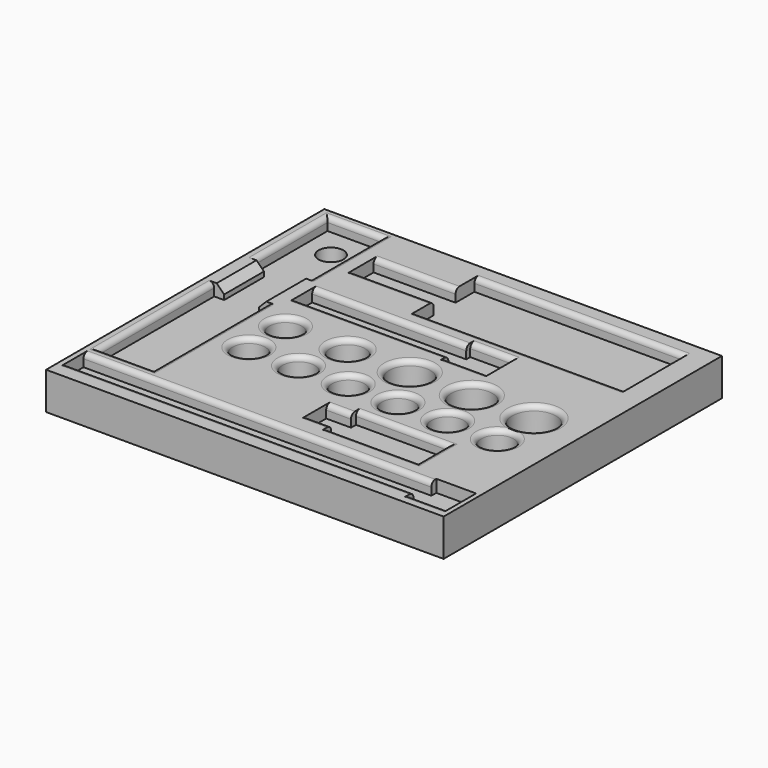
from build123d import *

# Parameters (mm, degrees)
F0_W          = 160
F0_H          = 140
F0_R          = 6.5
F0_R_2        = 7
F0_R_3        = 8.25
F0_R_4        = 8.75
F0_R_5        = 5
F1_DEPTH      = 1
F2_DEPTH      = 10
F3_DEPTH      = 15
F4_SIZE       = 3
F5_T1_DEPTH   = 37
F5_T3_DEPTH   = 58
F5_T5_DEPTH   = 22
F5_T7_DEPTH   = 145
F5_T9_DEPTH   = 16
F5_T11_DEPTH  = 85
F5_T13_DEPTH  = 38
F5_T15_DEPTH  = 18
F5_T17_DEPTH  = 67
F5_T19_DEPTH  = 37
F5_T21_DEPTH  = 15
F5_T23_DEPTH  = 15
F5_T51_DEPTH  = 27
F5_T56_DEPTH  = 42
F5_T64_DEPTH  = 42
F5_T69_DEPTH  = 27
F5_T76_DEPTH  = 63
F5_T80_DEPTH  = 27
F5_T87_DEPTH  = 27
F5_T92_DEPTH  = 63
F5_T99_DEPTH  = 42
F5_T103_DEPTH = 20
F5_T110_DEPTH = 20
F5_T114_DEPTH = 42


# Not quite as in the source:
# - a fillet or chamfer that OpenCascade refuses, or shapes differently, is made with other operations: its cross-section is extruded or revolved along the edge and cut away or added
# - a feature names something its author has since deleted; it is built from what else it names


with BuildPart() as f1:
    # F0 (on Top) → F1 (new body)
    with BuildSketch(Plane.XY):
        Rectangle(F0_W, F0_H)
        with Locations((-39.7392310202, -18.3150917292)):
            Circle(F0_R, mode=Mode.SUBTRACT)
        with Locations((-19.7392310202, -18.3150917292)):
            Circle(F0_R, mode=Mode.SUBTRACT)
        Polygon((78.1284613013, -51.3328099847), (78.1284613013, -65.3328099847), (62.1284613013, -65.3328099847), (62.1284613013, -62.8328099847), (-77.8715386987, -62.8328099847), (-77.8715386987, -53.8328099847), (62.1284613013, -53.8328099847), (62.1284613013, -51.3328099847), align=None, mode=Mode.SUBTRACT)
        Polygon((3.4841548279, -43.4470043983), (3.4841548279, -33.4470043983), (13.4841548279, -33.4470043983), (13.4841548279, -30.9470043983), (50.4841548279, -30.9470043983), (50.4841548279, -45.9470043983), (13.4841548279, -45.9470043983), (13.4841548279, -43.4470043983), align=None, mode=Mode.SUBTRACT)
        with Locations((0.2607689798, -18.3150917292)):
            Circle(F0_R, mode=Mode.SUBTRACT)
        with Locations((20.2607689798, -18.3150917292)):
            Circle(F0_R, mode=Mode.SUBTRACT)
        with Locations((40.2607689798, -18.3150917292)):
            Circle(F0_R, mode=Mode.SUBTRACT)
        with Locations((60.2607689798, -18.3150917292)):
            Circle(F0_R, mode=Mode.SUBTRACT)
        Polygon((-75.9079491794, 29.4701200724), (-75.9079491794, 66.4701200724), (-53.9079491794, 66.4701200724), (-53.9079491794, 29.4701200724), (-57.9079491794, 29.4701200724), (-57.9079491794, 9.4701200724), (-53.9079491794, 9.4701200724), (-53.9079491794, -48.5298799276), (-75.9079491794, -48.5298799276), (-75.9079491794, 9.4701200724), (-71.9079491794, 9.4701200724), (-71.9079491794, 29.4701200724), align=None, mode=Mode.SUBTRACT)
        with Locations((-39.6466106176, 0)):
            Circle(F0_R, mode=Mode.SUBTRACT)
        with Locations((-14.6466106176, 0)):
            Circle(F0_R_2, mode=Mode.SUBTRACT)
        Polygon((30.7263465822, 27.4683196438), (30.7263465822, 14.4683196438), (12.7263465822, 14.4683196438), (12.7263465822, 16.4683196438), (-49.2736534178, 16.4683196438), (-49.2736534178, 25.4683196438), (12.7263465822, 25.4683196438), (12.7263465822, 27.4683196438), align=None, mode=Mode.SUBTRACT)
        with Locations((10.3533893824, 0)):
            Circle(F0_R_3, mode=Mode.SUBTRACT)
        with Locations((35.3533893824, 0)):
            Circle(F0_R_3, mode=Mode.SUBTRACT)
        with Locations((60.3533893824, 0)):
            Circle(F0_R_4, mode=Mode.SUBTRACT)
        Polygon((71.00115427, 62.9950422049), (71.00115427, 32.9950422049), (-13.99884573, 32.9950422049), (-13.99884573, 42.4950422049), (-46.99884573, 42.4950422049), (-46.99884573, 53.4950422049), (-13.99884573, 53.4950422049), (-13.99884573, 62.9950422049), align=None, mode=Mode.SUBTRACT)
        Polygon((-13.99884573, 32.9950422049), (71.00115427, 32.9950422049), (71.00115427, 62.9950422049), (-13.99884573, 62.9950422049), (-13.99884573, 53.4950422049), (-46.99884573, 53.4950422049), (-46.99884573, 42.4950422049), (-13.99884573, 42.4950422049), align=None)
        Polygon((-53.9079491794, 66.4701200724), (-75.9079491794, 66.4701200724), (-75.9079491794, 29.4701200724), (-71.9079491794, 29.4701200724), (-71.9079491794, 9.4701200724), (-75.9079491794, 9.4701200724), (-75.9079491794, -48.5298799276), (-53.9079491794, -48.5298799276), (-53.9079491794, 9.4701200724), (-57.9079491794, 9.4701200724), (-57.9079491794, 29.4701200724), (-53.9079491794, 29.4701200724), align=None)
        with Locations((-64.9079491794, 54.4701200724)):
            Circle(F0_R_5, mode=Mode.SUBTRACT)
        Polygon((62.1284613013, -65.3328099847), (78.1284613013, -65.3328099847), (78.1284613013, -51.3328099847), (62.1284613013, -51.3328099847), (62.1284613013, -53.8328099847), (-77.8715386987, -53.8328099847), (-77.8715386987, -62.8328099847), (62.1284613013, -62.8328099847), align=None)
        Polygon((12.7263465822, 14.4683196438), (30.7263465822, 14.4683196438), (30.7263465822, 27.4683196438), (12.7263465822, 27.4683196438), (12.7263465822, 25.4683196438), (-49.2736534178, 25.4683196438), (-49.2736534178, 16.4683196438), (12.7263465822, 16.4683196438), align=None)
        Polygon((13.4841548279, -33.4470043983), (3.4841548279, -33.4470043983), (3.4841548279, -43.4470043983), (13.4841548279, -43.4470043983), (13.4841548279, -45.9470043983), (50.4841548279, -45.9470043983), (50.4841548279, -30.9470043983), (13.4841548279, -30.9470043983), align=None)
        with Locations((60.3533893824, 0)):
            Circle(F0_R_4)
        with Locations((10.3533893824, 0)):
            Circle(F0_R_3)
        with Locations((35.3533893824, 0)):
            Circle(F0_R_3)
        with Locations((-14.6466106176, 0)):
            Circle(F0_R_2)
        with Locations((-39.6466106176, 0)):
            Circle(F0_R)
        with Locations((-39.7392310202, -18.3150917292)):
            Circle(F0_R)
        with Locations((-19.7392310202, -18.3150917292)):
            Circle(F0_R)
        with Locations((0.2607689798, -18.3150917292)):
            Circle(F0_R)
        with Locations((20.2607689798, -18.3150917292)):
            Circle(F0_R)
        with Locations((40.2607689798, -18.3150917292)):
            Circle(F0_R)
        with Locations((60.2607689798, -18.3150917292)):
            Circle(F0_R)
        with Locations((-64.9079491794, 54.4701200724)):
            Circle(F0_R_5)
    extrude(amount=F1_DEPTH)

    # F0 (on Top) → F2 (join)
    with BuildSketch(Plane.XY):
        Rectangle(F0_W, F0_H)
        with Locations((-39.7392310202, -18.3150917292)):
            Circle(F0_R, mode=Mode.SUBTRACT)
        with Locations((-19.7392310202, -18.3150917292)):
            Circle(F0_R, mode=Mode.SUBTRACT)
        Polygon((78.1284613013, -51.3328099847), (78.1284613013, -65.3328099847), (62.1284613013, -65.3328099847), (62.1284613013, -62.8328099847), (-77.8715386987, -62.8328099847), (-77.8715386987, -53.8328099847), (62.1284613013, -53.8328099847), (62.1284613013, -51.3328099847), align=None, mode=Mode.SUBTRACT)
        Polygon((3.4841548279, -43.4470043983), (3.4841548279, -33.4470043983), (13.4841548279, -33.4470043983), (13.4841548279, -30.9470043983), (50.4841548279, -30.9470043983), (50.4841548279, -45.9470043983), (13.4841548279, -45.9470043983), (13.4841548279, -43.4470043983), align=None, mode=Mode.SUBTRACT)
        with Locations((0.2607689798, -18.3150917292)):
            Circle(F0_R, mode=Mode.SUBTRACT)
        with Locations((20.2607689798, -18.3150917292)):
            Circle(F0_R, mode=Mode.SUBTRACT)
        with Locations((40.2607689798, -18.3150917292)):
            Circle(F0_R, mode=Mode.SUBTRACT)
        with Locations((60.2607689798, -18.3150917292)):
            Circle(F0_R, mode=Mode.SUBTRACT)
        Polygon((-75.9079491794, 29.4701200724), (-75.9079491794, 66.4701200724), (-53.9079491794, 66.4701200724), (-53.9079491794, 29.4701200724), (-57.9079491794, 29.4701200724), (-57.9079491794, 9.4701200724), (-53.9079491794, 9.4701200724), (-53.9079491794, -48.5298799276), (-75.9079491794, -48.5298799276), (-75.9079491794, 9.4701200724), (-71.9079491794, 9.4701200724), (-71.9079491794, 29.4701200724), align=None, mode=Mode.SUBTRACT)
        with Locations((-39.6466106176, 0)):
            Circle(F0_R, mode=Mode.SUBTRACT)
        with Locations((-14.6466106176, 0)):
            Circle(F0_R_2, mode=Mode.SUBTRACT)
        Polygon((30.7263465822, 27.4683196438), (30.7263465822, 14.4683196438), (12.7263465822, 14.4683196438), (12.7263465822, 16.4683196438), (-49.2736534178, 16.4683196438), (-49.2736534178, 25.4683196438), (12.7263465822, 25.4683196438), (12.7263465822, 27.4683196438), align=None, mode=Mode.SUBTRACT)
        with Locations((10.3533893824, 0)):
            Circle(F0_R_3, mode=Mode.SUBTRACT)
        with Locations((35.3533893824, 0)):
            Circle(F0_R_3, mode=Mode.SUBTRACT)
        with Locations((60.3533893824, 0)):
            Circle(F0_R_4, mode=Mode.SUBTRACT)
        Polygon((71.00115427, 62.9950422049), (71.00115427, 32.9950422049), (-13.99884573, 32.9950422049), (-13.99884573, 42.4950422049), (-46.99884573, 42.4950422049), (-46.99884573, 53.4950422049), (-13.99884573, 53.4950422049), (-13.99884573, 62.9950422049), align=None, mode=Mode.SUBTRACT)
        Polygon((62.1284613013, -65.3328099847), (78.1284613013, -65.3328099847), (78.1284613013, -51.3328099847), (62.1284613013, -51.3328099847), (62.1284613013, -53.8328099847), (-77.8715386987, -53.8328099847), (-77.8715386987, -62.8328099847), (62.1284613013, -62.8328099847), align=None)
        Polygon((-53.9079491794, 66.4701200724), (-75.9079491794, 66.4701200724), (-75.9079491794, 29.4701200724), (-71.9079491794, 29.4701200724), (-71.9079491794, 9.4701200724), (-75.9079491794, 9.4701200724), (-75.9079491794, -48.5298799276), (-53.9079491794, -48.5298799276), (-53.9079491794, 9.4701200724), (-57.9079491794, 9.4701200724), (-57.9079491794, 29.4701200724), (-53.9079491794, 29.4701200724), align=None)
        with Locations((-64.9079491794, 54.4701200724)):
            Circle(F0_R_5, mode=Mode.SUBTRACT)
        Polygon((12.7263465822, 14.4683196438), (30.7263465822, 14.4683196438), (30.7263465822, 27.4683196438), (12.7263465822, 27.4683196438), (12.7263465822, 25.4683196438), (-49.2736534178, 25.4683196438), (-49.2736534178, 16.4683196438), (12.7263465822, 16.4683196438), align=None)
        Polygon((13.4841548279, -33.4470043983), (3.4841548279, -33.4470043983), (3.4841548279, -43.4470043983), (13.4841548279, -43.4470043983), (13.4841548279, -45.9470043983), (50.4841548279, -45.9470043983), (50.4841548279, -30.9470043983), (13.4841548279, -30.9470043983), align=None)
        Polygon((-13.99884573, 32.9950422049), (71.00115427, 32.9950422049), (71.00115427, 62.9950422049), (-13.99884573, 62.9950422049), (-13.99884573, 53.4950422049), (-46.99884573, 53.4950422049), (-46.99884573, 42.4950422049), (-13.99884573, 42.4950422049), align=None)
    extrude(amount=F2_DEPTH)

    # F0 (on Top) → F3 (join)
    with BuildSketch(Plane.XY):
        Rectangle(F0_W, F0_H)
        with Locations((-39.7392310202, -18.3150917292)):
            Circle(F0_R, mode=Mode.SUBTRACT)
        with Locations((-19.7392310202, -18.3150917292)):
            Circle(F0_R, mode=Mode.SUBTRACT)
        Polygon((78.1284613013, -51.3328099847), (78.1284613013, -65.3328099847), (62.1284613013, -65.3328099847), (62.1284613013, -62.8328099847), (-77.8715386987, -62.8328099847), (-77.8715386987, -53.8328099847), (62.1284613013, -53.8328099847), (62.1284613013, -51.3328099847), align=None, mode=Mode.SUBTRACT)
        Polygon((3.4841548279, -43.4470043983), (3.4841548279, -33.4470043983), (13.4841548279, -33.4470043983), (13.4841548279, -30.9470043983), (50.4841548279, -30.9470043983), (50.4841548279, -45.9470043983), (13.4841548279, -45.9470043983), (13.4841548279, -43.4470043983), align=None, mode=Mode.SUBTRACT)
        with Locations((0.2607689798, -18.3150917292)):
            Circle(F0_R, mode=Mode.SUBTRACT)
        with Locations((20.2607689798, -18.3150917292)):
            Circle(F0_R, mode=Mode.SUBTRACT)
        with Locations((40.2607689798, -18.3150917292)):
            Circle(F0_R, mode=Mode.SUBTRACT)
        with Locations((60.2607689798, -18.3150917292)):
            Circle(F0_R, mode=Mode.SUBTRACT)
        Polygon((-75.9079491794, 29.4701200724), (-75.9079491794, 66.4701200724), (-53.9079491794, 66.4701200724), (-53.9079491794, 29.4701200724), (-57.9079491794, 29.4701200724), (-57.9079491794, 9.4701200724), (-53.9079491794, 9.4701200724), (-53.9079491794, -48.5298799276), (-75.9079491794, -48.5298799276), (-75.9079491794, 9.4701200724), (-71.9079491794, 9.4701200724), (-71.9079491794, 29.4701200724), align=None, mode=Mode.SUBTRACT)
        with Locations((-39.6466106176, 0)):
            Circle(F0_R, mode=Mode.SUBTRACT)
        with Locations((-14.6466106176, 0)):
            Circle(F0_R_2, mode=Mode.SUBTRACT)
        Polygon((30.7263465822, 27.4683196438), (30.7263465822, 14.4683196438), (12.7263465822, 14.4683196438), (12.7263465822, 16.4683196438), (-49.2736534178, 16.4683196438), (-49.2736534178, 25.4683196438), (12.7263465822, 25.4683196438), (12.7263465822, 27.4683196438), align=None, mode=Mode.SUBTRACT)
        with Locations((10.3533893824, 0)):
            Circle(F0_R_3, mode=Mode.SUBTRACT)
        with Locations((35.3533893824, 0)):
            Circle(F0_R_3, mode=Mode.SUBTRACT)
        with Locations((60.3533893824, 0)):
            Circle(F0_R_4, mode=Mode.SUBTRACT)
        Polygon((71.00115427, 62.9950422049), (71.00115427, 32.9950422049), (-13.99884573, 32.9950422049), (-13.99884573, 42.4950422049), (-46.99884573, 42.4950422049), (-46.99884573, 53.4950422049), (-13.99884573, 53.4950422049), (-13.99884573, 62.9950422049), align=None, mode=Mode.SUBTRACT)
    extrude(amount=F3_DEPTH)

    # F4
    f4_edges = [f1.edges().sort_by_distance(p)[0] for p in [
        (-57.907949, 19.47012, 15),
        (-71.907949, 19.47012, 15),
    ]]
    chamfer(f4_edges, length=F4_SIZE)

    # F5: fillet of radius 2 on 33 edges, made by hand

    # F5_s2 → F5_t1 (cut)
    with BuildSketch(Plane.XZ.offset(-66.4701200724)):
        with BuildLine():
            ThreePointArc((-77.9079491794, 15), (-76.493735617, 14.4142135624), (-75.9079491794, 13))
            Line((-75.9079491794, 13), (-75.9079491794, 15))
            Line((-75.9079491794, 15), (-77.9079491794, 15))
        make_face()
        with BuildLine():
            ThreePointArc((-51.9079491794, 15), (-53.3221627418, 14.4142135624), (-53.9079491794, 13))
            Line((-53.9079491794, 13), (-53.9079491794, 15))
            Line((-53.9079491794, 15), (-51.9079491794, 15))
        make_face()
    extrude(amount=F5_T1_DEPTH, mode=Mode.SUBTRACT)

    # F5_s4 → F5_t3 (cut)
    with BuildSketch(Plane.XZ.offset(-9.4701200724)):
        with BuildLine():
            ThreePointArc((-51.9079491794, 15), (-53.3221627418, 14.4142135624), (-53.9079491794, 13))
            Line((-53.9079491794, 13), (-53.9079491794, 15))
            Line((-53.9079491794, 15), (-51.9079491794, 15))
        make_face()
        with BuildLine():
            ThreePointArc((-77.9079491794, 15), (-76.493735617, 14.4142135624), (-75.9079491794, 13))
            Line((-75.9079491794, 13), (-75.9079491794, 15))
            Line((-75.9079491794, 15), (-77.9079491794, 15))
        make_face()
    extrude(amount=F5_T3_DEPTH, mode=Mode.SUBTRACT)

    # F5_s6 → F5_t5 (cut)
    with BuildSketch(Plane.YZ.offset(-75.9079491794)):
        with BuildLine():
            ThreePointArc((-50.5298799276, 15), (-49.1156663653, 14.4142135624), (-48.5298799276, 13))
            Line((-48.5298799276, 13), (-48.5298799276, 15))
            Line((-48.5298799276, 15), (-50.5298799276, 15))
        make_face()
        with BuildLine():
            ThreePointArc((68.4701200724, 15), (67.05590651, 14.4142135624), (66.4701200724, 13))
            Line((66.4701200724, 13), (66.4701200724, 15))
            Line((66.4701200724, 15), (68.4701200724, 15))
        make_face()
    extrude(amount=F5_T5_DEPTH, mode=Mode.SUBTRACT)

    # F5_s8 → F5_t7 (cut)
    with BuildSketch(Plane.YZ.offset(-77.8715386987)):
        with BuildLine():
            ThreePointArc((-64.8328099847, 15), (-63.4185964223, 14.4142135624), (-62.8328099847, 13))
            Line((-62.8328099847, 13), (-62.8328099847, 15))
            Line((-62.8328099847, 15), (-64.8328099847, 15))
        make_face()
        with BuildLine():
            ThreePointArc((-51.8328099847, 15), (-53.2470235471, 14.4142135624), (-53.8328099847, 13))
            Line((-53.8328099847, 13), (-53.8328099847, 15))
            Line((-53.8328099847, 15), (-51.8328099847, 15))
        make_face()
    extrude(amount=F5_T7_DEPTH, mode=Mode.SUBTRACT)

    # F5_s10 → F5_t9 (cut)
    with BuildSketch(Plane.YZ.offset(62.1284613013)):
        with BuildLine():
            ThreePointArc((-67.3328099847, 15), (-65.9185964223, 14.4142135624), (-65.3328099847, 13))
            Line((-65.3328099847, 13), (-65.3328099847, 15))
            Line((-65.3328099847, 15), (-67.3328099847, 15))
        make_face()
    extrude(amount=F5_T9_DEPTH, mode=Mode.SUBTRACT)

    # F5_s12 → F5_t11 (cut)
    with BuildSketch(Plane.YZ.offset(-13.99884573)):
        with BuildLine():
            ThreePointArc((64.9950422049, 15), (63.5808286425, 14.4142135624), (62.9950422049, 13))
            Line((62.9950422049, 13), (62.9950422049, 15))
            Line((62.9950422049, 15), (64.9950422049, 15))
        make_face()
        with BuildLine():
            ThreePointArc((30.9950422049, 15), (32.4092557672, 14.4142135624), (32.9950422049, 13))
            Line((32.9950422049, 13), (32.9950422049, 15))
            Line((32.9950422049, 15), (30.9950422049, 15))
        make_face()
    extrude(amount=F5_T11_DEPTH, mode=Mode.SUBTRACT)

    # F5_s14 → F5_t13 (cut)
    with BuildSketch(Plane.YZ.offset(-46.99884573)):
        with BuildLine():
            ThreePointArc((40.4950422049, 15), (41.9092557672, 14.4142135624), (42.4950422049, 13))
            Line((42.4950422049, 13), (42.4950422049, 15))
            Line((42.4950422049, 15), (40.4950422049, 15))
        make_face()
        with BuildLine():
            ThreePointArc((55.4950422049, 15), (54.0808286425, 14.4142135624), (53.4950422049, 13))
            Line((53.4950422049, 13), (53.4950422049, 15))
            Line((53.4950422049, 15), (55.4950422049, 15))
        make_face()
    extrude(amount=F5_T13_DEPTH, mode=Mode.SUBTRACT)

    # F5_s16 → F5_t15 (cut)
    with BuildSketch(Plane.YZ.offset(12.7263465822)):
        with BuildLine():
            ThreePointArc((29.4683196438, 15), (28.0541060814, 14.4142135624), (27.4683196438, 13))
            Line((27.4683196438, 13), (27.4683196438, 15))
            Line((27.4683196438, 15), (29.4683196438, 15))
        make_face()
        with BuildLine():
            ThreePointArc((12.4683196438, 15), (13.8825332061, 14.4142135624), (14.4683196438, 13))
            Line((14.4683196438, 13), (14.4683196438, 15))
            Line((14.4683196438, 15), (12.4683196438, 15))
        make_face()
    extrude(amount=F5_T15_DEPTH, mode=Mode.SUBTRACT)

    # F5_s18 → F5_t17 (cut)
    with BuildSketch(Plane.YZ.offset(-49.2736534178)):
        with BuildLine():
            ThreePointArc((14.4683196438, 15), (15.8825332061, 14.4142135624), (16.4683196438, 13))
            Line((16.4683196438, 13), (16.4683196438, 15))
            Line((16.4683196438, 15), (14.4683196438, 15))
        make_face()
        with BuildLine():
            ThreePointArc((27.4683196438, 15), (26.0541060814, 14.4142135624), (25.4683196438, 13))
            Line((25.4683196438, 13), (25.4683196438, 15))
            Line((25.4683196438, 15), (27.4683196438, 15))
        make_face()
    extrude(amount=F5_T17_DEPTH, mode=Mode.SUBTRACT)

    # F5_s20 → F5_t19 (cut)
    with BuildSketch(Plane.YZ.offset(13.4841548279)):
        with BuildLine():
            ThreePointArc((-28.9470043983, 15), (-30.3612179607, 14.4142135624), (-30.9470043983, 13))
            Line((-30.9470043983, 13), (-30.9470043983, 15))
            Line((-30.9470043983, 15), (-28.9470043983, 15))
        make_face()
        with BuildLine():
            ThreePointArc((-47.9470043983, 15), (-46.532790836, 14.4142135624), (-45.9470043983, 13))
            Line((-45.9470043983, 13), (-45.9470043983, 15))
            Line((-45.9470043983, 15), (-47.9470043983, 15))
        make_face()
    extrude(amount=F5_T19_DEPTH, mode=Mode.SUBTRACT)

    # F5_s22 → F5_t21 (cut)
    with BuildSketch(Plane.YZ.offset(3.4841548279)):
        with BuildLine():
            ThreePointArc((-45.4470043983, 15), (-44.032790836, 14.4142135624), (-43.4470043983, 13))
            Line((-43.4470043983, 13), (-43.4470043983, 15))
            Line((-43.4470043983, 15), (-45.4470043983, 15))
        make_face()
        with BuildLine():
            ThreePointArc((-31.4470043983, 15), (-32.8612179607, 14.4142135624), (-33.4470043983, 13))
            Line((-33.4470043983, 13), (-33.4470043983, 15))
            Line((-33.4470043983, 15), (-31.4470043983, 15))
        make_face()
    extrude(amount=F5_T21_DEPTH, mode=Mode.SUBTRACT)

    # F5_s24 → F5_t23 (cut)
    with BuildSketch(Plane.XZ.offset(30.9470043983)):
        with BuildLine():
            ThreePointArc((52.4841548279, 15), (51.0699412655, 14.4142135624), (50.4841548279, 13))
            Line((50.4841548279, 13), (50.4841548279, 15))
            Line((50.4841548279, 15), (52.4841548279, 15))
        make_face()
    extrude(amount=F5_T23_DEPTH, mode=Mode.SUBTRACT)

    # F5_s25 → F5_t26 (revolve, cut)
    with BuildSketch(Plane.XZ):
        with BuildLine():
            ThreePointArc((-31.1466106176, 15), (-32.56082418, 14.4142135624), (-33.1466106176, 13))
            Line((-33.1466106176, 13), (-33.1466106176, 15))
            Line((-33.1466106176, 15), (-31.1466106176, 15))
        make_face()
    revolve(axis=Axis((-39.6466106176, 0, 15), (0, 0, 1)), mode=Mode.SUBTRACT)

    # F5_s27 → F5_t28 (revolve, cut)
    with BuildSketch(Plane.XZ):
        with BuildLine():
            ThreePointArc((-5.6466106176, 15), (-7.06082418, 14.4142135624), (-7.6466106176, 13))
            Line((-7.6466106176, 13), (-7.6466106176, 15))
            Line((-7.6466106176, 15), (-5.6466106176, 15))
        make_face()
    revolve(axis=Axis((-14.6466106176, 0, 15), (0, 0, 1)), mode=Mode.SUBTRACT)

    # F5_s29 → F5_t30 (revolve, cut)
    with BuildSketch(Plane.XZ):
        with BuildLine():
            ThreePointArc((20.6033893824, 15), (19.18917582, 14.4142135624), (18.6033893824, 13))
            Line((18.6033893824, 13), (18.6033893824, 15))
            Line((18.6033893824, 15), (20.6033893824, 15))
        make_face()
    revolve(axis=Axis((10.3533893824, 0, 15), (0, 0, 1)), mode=Mode.SUBTRACT)

    # F5_s31 → F5_t32 (revolve, cut)
    with BuildSketch(Plane.XZ):
        with BuildLine():
            ThreePointArc((45.6033893824, 15), (44.18917582, 14.4142135624), (43.6033893824, 13))
            Line((43.6033893824, 13), (43.6033893824, 15))
            Line((43.6033893824, 15), (45.6033893824, 15))
        make_face()
    revolve(axis=Axis((35.3533893824, 0, 15), (0, 0, 1)), mode=Mode.SUBTRACT)

    # F5_s33 → F5_t34 (revolve, cut)
    with BuildSketch(Plane.XZ):
        with BuildLine():
            ThreePointArc((71.1033893824, 15), (69.68917582, 14.4142135624), (69.1033893824, 13))
            Line((69.1033893824, 13), (69.1033893824, 15))
            Line((69.1033893824, 15), (71.1033893824, 15))
        make_face()
    revolve(axis=Axis((60.3533893824, 0, 15), (0, 0, 1)), mode=Mode.SUBTRACT)

    # F5_s35 → F5_t36 (revolve, cut)
    with BuildSketch(Plane.XZ.offset(18.3150917292)):
        with BuildLine():
            ThreePointArc((68.7607689798, 15), (67.3465554174, 14.4142135624), (66.7607689798, 13))
            Line((66.7607689798, 13), (66.7607689798, 15))
            Line((66.7607689798, 15), (68.7607689798, 15))
        make_face()
    revolve(axis=Axis((60.2607689798, -18.3150917292, 15), (0, 0, 1)), mode=Mode.SUBTRACT)

    # F5_s37 → F5_t38 (revolve, cut)
    with BuildSketch(Plane.XZ.offset(18.3150917292)):
        with BuildLine():
            ThreePointArc((48.7607689798, 15), (47.3465554174, 14.4142135624), (46.7607689798, 13))
            Line((46.7607689798, 13), (46.7607689798, 15))
            Line((46.7607689798, 15), (48.7607689798, 15))
        make_face()
    revolve(axis=Axis((40.2607689798, -18.3150917292, 15), (0, 0, 1)), mode=Mode.SUBTRACT)

    # F5_s39 → F5_t40 (revolve, cut)
    with BuildSketch(Plane.XZ.offset(18.3150917292)):
        with BuildLine():
            ThreePointArc((28.7607689798, 15), (27.3465554174, 14.4142135624), (26.7607689798, 13))
            Line((26.7607689798, 13), (26.7607689798, 15))
            Line((26.7607689798, 15), (28.7607689798, 15))
        make_face()
    revolve(axis=Axis((20.2607689798, -18.3150917292, 15), (0, 0, 1)), mode=Mode.SUBTRACT)

    # F5_s41 → F5_t42 (revolve, cut)
    with BuildSketch(Plane.XZ.offset(18.3150917292)):
        with BuildLine():
            ThreePointArc((8.7607689798, 15), (7.3465554174, 14.4142135624), (6.7607689798, 13))
            Line((6.7607689798, 13), (6.7607689798, 15))
            Line((6.7607689798, 15), (8.7607689798, 15))
        make_face()
    revolve(axis=Axis((0.2607689798, -18.3150917292, 15), (0, 0, 1)), mode=Mode.SUBTRACT)

    # F5_s43 → F5_t44 (revolve, cut)
    with BuildSketch(Plane.XZ.offset(18.3150917292)):
        with BuildLine():
            ThreePointArc((-11.2392310202, 15), (-12.6534445826, 14.4142135624), (-13.2392310202, 13))
            Line((-13.2392310202, 13), (-13.2392310202, 15))
            Line((-13.2392310202, 15), (-11.2392310202, 15))
        make_face()
    revolve(axis=Axis((-19.7392310202, -18.3150917292, 15), (0, 0, 1)), mode=Mode.SUBTRACT)

    # F5_s45 → F5_t46 (revolve, cut)
    with BuildSketch(Plane.XZ.offset(18.3150917292)):
        with BuildLine():
            ThreePointArc((-31.2392310202, 15), (-32.6534445826, 14.4142135624), (-33.2392310202, 13))
            Line((-33.2392310202, 13), (-33.2392310202, 15))
            Line((-33.2392310202, 15), (-31.2392310202, 15))
        make_face()
    revolve(axis=Axis((-39.7392310202, -18.3150917292, 15), (0, 0, 1)), mode=Mode.SUBTRACT)


with BuildPart() as f5_tool49:
    # F5_s50 → F5_t51 (new body)
    with BuildSketch(Plane.YZ.offset(-80.9079491794)):
        with BuildLine():
            ThreePointArc((68.4701200724, 15), (67.05590651, 14.4142135624), (66.4701200724, 13))
            Line((66.4701200724, 13), (66.4701200724, 15))
            Line((66.4701200724, 15), (68.4701200724, 15))
        make_face()
    extrude(amount=F5_T51_DEPTH)

    split(bisect_by=Plane.YZ.offset(-75.9079491794), keep=Keep.BOTTOM)

    split(bisect_by=Plane.YZ.offset(-80), keep=Keep.TOP)


with BuildPart() as f5_tool54:
    # F5_s55 → F5_t56 (new body)
    with BuildSketch(Plane.XZ.offset(-29.4701200724)):
        with BuildLine():
            ThreePointArc((-77.9079491794, 15), (-76.493735617, 14.4142135624), (-75.9079491794, 13))
            Line((-75.9079491794, 13), (-75.9079491794, 15))
            Line((-75.9079491794, 15), (-77.9079491794, 15))
        make_face()
    extrude(amount=-F5_T56_DEPTH)

    split(bisect_by=Plane.XZ.offset(-66.4701200724), keep=Keep.BOTTOM)

    split(bisect_by=Plane.XZ.offset(-70), keep=Keep.TOP)


with BuildPart() as f5_tool49_1:
    add(f5_tool49.part)

    # F5_t59: intersect F5_tool54
    add(f5_tool54.part, mode=Mode.INTERSECT)


with BuildPart() as f1_1:
    add(f1.part)

    # F5_t47: cut F5_tool49
    add(f5_tool49_1.part, mode=Mode.SUBTRACT)


with BuildPart() as f5_tool62:
    # F5_s63 → F5_t64 (new body)
    with BuildSketch(Plane.XZ.offset(-71.4701200724)):
        with BuildLine():
            ThreePointArc((-51.9079491794, 15), (-53.3221627418, 14.4142135624), (-53.9079491794, 13))
            Line((-53.9079491794, 13), (-53.9079491794, 15))
            Line((-53.9079491794, 15), (-51.9079491794, 15))
        make_face()
    extrude(amount=F5_T64_DEPTH)

    split(bisect_by=Plane.XZ.offset(-66.4701200724), keep=Keep.BOTTOM)

    split(bisect_by=Plane.XZ.offset(-70), keep=Keep.TOP)


with BuildPart() as f5_tool67:
    # F5_s68 → F5_t69 (new body)
    with BuildSketch(Plane.YZ.offset(-75.9079491794)):
        with BuildLine():
            ThreePointArc((68.4701200724, 15), (67.05590651, 14.4142135624), (66.4701200724, 13))
            Line((66.4701200724, 13), (66.4701200724, 15))
            Line((66.4701200724, 15), (68.4701200724, 15))
        make_face()
    extrude(amount=F5_T69_DEPTH)

    split(bisect_by=Plane.YZ.offset(-53.9079491794), keep=Keep.TOP)


with BuildPart() as f5_tool62_1:
    add(f5_tool62.part)

    # F5_t71: intersect F5_tool67
    add(f5_tool67.part, mode=Mode.INTERSECT)


with BuildPart() as f1_2:
    add(f1_1.part)

    # F5_t60: cut F5_tool62
    add(f5_tool62_1.part, mode=Mode.SUBTRACT)


with BuildPart() as f5_tool74:
    # F5_s75 → F5_t76 (new body)
    with BuildSketch(Plane.XZ.offset(-9.4701200724)):
        with BuildLine():
            ThreePointArc((-51.9079491794, 15), (-53.3221627418, 14.4142135624), (-53.9079491794, 13))
            Line((-53.9079491794, 13), (-53.9079491794, 15))
            Line((-53.9079491794, 15), (-51.9079491794, 15))
        make_face()
    extrude(amount=F5_T76_DEPTH)

    split(bisect_by=Plane.XZ.offset(48.5298799276), keep=Keep.TOP)


with BuildPart() as f5_tool78:
    # F5_s79 → F5_t80 (new body)
    with BuildSketch(Plane.YZ.offset(-48.9079491794)):
        with BuildLine():
            ThreePointArc((-50.5298799276, 15), (-49.1156663653, 14.4142135624), (-48.5298799276, 13))
            Line((-48.5298799276, 13), (-48.5298799276, 15))
            Line((-48.5298799276, 15), (-50.5298799276, 15))
        make_face()
    extrude(amount=-F5_T80_DEPTH)

    split(bisect_by=Plane.YZ.offset(-53.9079491794), keep=Keep.TOP)


with BuildPart() as f5_tool74_1:
    add(f5_tool74.part)

    # F5_t82: intersect F5_tool78
    add(f5_tool78.part, mode=Mode.INTERSECT)


with BuildPart() as f1_3:
    add(f1_2.part)

    # F5_t72: cut F5_tool74
    add(f5_tool74_1.part, mode=Mode.SUBTRACT)


with BuildPart() as f5_tool85:
    # F5_s86 → F5_t87 (new body)
    with BuildSketch(Plane.YZ.offset(-53.9079491794)):
        with BuildLine():
            ThreePointArc((-50.5298799276, 15), (-49.1156663653, 14.4142135624), (-48.5298799276, 13))
            Line((-48.5298799276, 13), (-48.5298799276, 15))
            Line((-48.5298799276, 15), (-50.5298799276, 15))
        make_face()
    extrude(amount=-F5_T87_DEPTH)

    split(bisect_by=Plane.YZ.offset(-75.9079491794), keep=Keep.BOTTOM)

    split(bisect_by=Plane.YZ.offset(-80), keep=Keep.TOP)


with BuildPart() as f5_tool90:
    # F5_s91 → F5_t92 (new body)
    with BuildSketch(Plane.XZ.offset(53.5298799276)):
        with BuildLine():
            ThreePointArc((-77.9079491794, 15), (-76.493735617, 14.4142135624), (-75.9079491794, 13))
            Line((-75.9079491794, 13), (-75.9079491794, 15))
            Line((-75.9079491794, 15), (-77.9079491794, 15))
        make_face()
    extrude(amount=-F5_T92_DEPTH)

    split(bisect_by=Plane.XZ.offset(48.5298799276), keep=Keep.TOP)


with BuildPart() as f5_tool85_1:
    add(f5_tool85.part)

    # F5_t94: intersect F5_tool90
    add(f5_tool90.part, mode=Mode.INTERSECT)


with BuildPart() as f1_4:
    add(f1_3.part)

    # F5_t83: cut F5_tool85
    add(f5_tool85_1.part, mode=Mode.SUBTRACT)


with BuildPart() as f5_tool97:
    # F5_s98 → F5_t99 (new body)
    with BuildSketch(Plane.YZ.offset(13.4841548279)):
        with BuildLine():
            ThreePointArc((-28.9470043983, 15), (-30.3612179607, 14.4142135624), (-30.9470043983, 13))
            Line((-30.9470043983, 13), (-30.9470043983, 15))
            Line((-30.9470043983, 15), (-28.9470043983, 15))
        make_face()
    extrude(amount=F5_T99_DEPTH)

    split(bisect_by=Plane.YZ.offset(50.4841548279), keep=Keep.TOP)


with BuildPart() as f5_tool101:
    # F5_s102 → F5_t103 (new body)
    with BuildSketch(Plane.XZ.offset(25.9470043983)):
        with BuildLine():
            ThreePointArc((52.4841548279, 15), (51.0699412655, 14.4142135624), (50.4841548279, 13))
            Line((50.4841548279, 13), (50.4841548279, 15))
            Line((50.4841548279, 15), (52.4841548279, 15))
        make_face()
    extrude(amount=F5_T103_DEPTH)

    split(bisect_by=Plane.XZ.offset(30.9470043983), keep=Keep.BOTTOM)


with BuildPart() as f5_tool97_1:
    add(f5_tool97.part)

    # F5_t105: intersect F5_tool101
    add(f5_tool101.part, mode=Mode.INTERSECT)


with BuildPart() as f1_5:
    add(f1_4.part)

    # F5_t95: cut F5_tool97
    add(f5_tool97_1.part, mode=Mode.SUBTRACT)


with BuildPart() as f5_tool108:
    # F5_s109 → F5_t110 (new body)
    with BuildSketch(Plane.XZ.offset(30.9470043983)):
        with BuildLine():
            ThreePointArc((52.4841548279, 15), (51.0699412655, 14.4142135624), (50.4841548279, 13))
            Line((50.4841548279, 13), (50.4841548279, 15))
            Line((50.4841548279, 15), (52.4841548279, 15))
        make_face()
    extrude(amount=F5_T110_DEPTH)

    split(bisect_by=Plane.XZ.offset(45.9470043983), keep=Keep.TOP)


with BuildPart() as f5_tool112:
    # F5_s113 → F5_t114 (new body)
    with BuildSketch(Plane.YZ.offset(55.4841548279)):
        with BuildLine():
            ThreePointArc((-47.9470043983, 15), (-46.532790836, 14.4142135624), (-45.9470043983, 13))
            Line((-45.9470043983, 13), (-45.9470043983, 15))
            Line((-45.9470043983, 15), (-47.9470043983, 15))
        make_face()
    extrude(amount=-F5_T114_DEPTH)

    split(bisect_by=Plane.YZ.offset(50.4841548279), keep=Keep.TOP)


with BuildPart() as f5_tool108_1:
    add(f5_tool108.part)

    # F5_t116: intersect F5_tool112
    add(f5_tool112.part, mode=Mode.INTERSECT)


with BuildPart() as f1_6:
    add(f1_5.part)

    # F5_t106: cut F5_tool108
    add(f5_tool108_1.part, mode=Mode.SUBTRACT)


solid = f1_6.part
